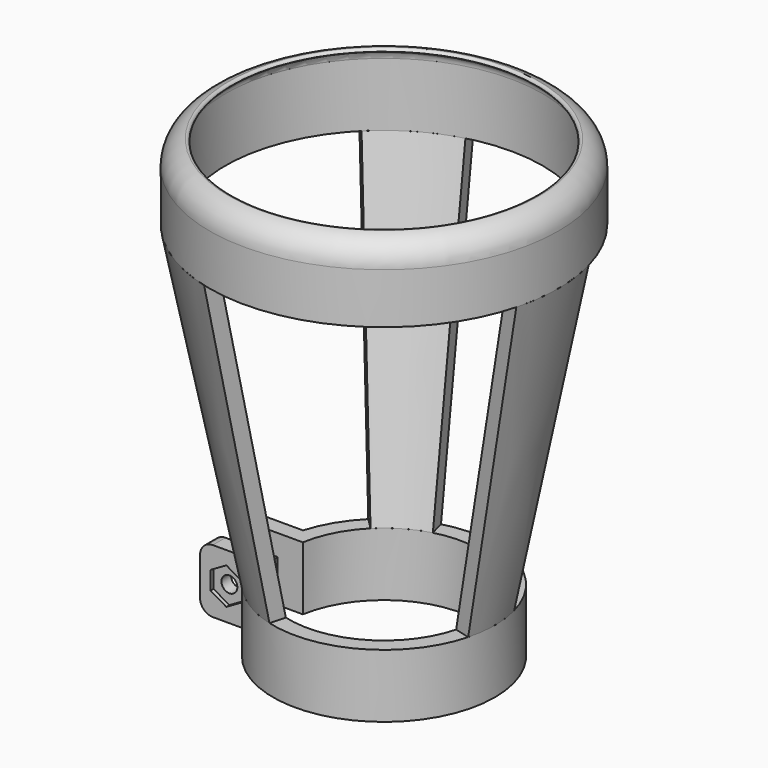
from build123d import *

# Parameters (mm, degrees)
F0_W           = 3.175
F0_H           = 12.7
F1_ANGLE_BACK  = 15
F1_ANGLE       = 30
F0_W_2         = 4.4764786097
F0_H_2         = 0.6337500702
F4_COUNT       = 3
F4_ANGLE       = 240
F0_W_3         = 7.0289915919
F5_DEPTH       = 6.35
F6_DEPTH       = 3.175
F8_D           = 3.175
F8_CBORE_D     = 6.35
F8_CBORE_DEPTH = 0.508
F9_R           = 1.5875
F10_DEPTH      = 0.762
F12_R          = 0.508


# Not quite as in the source:
# - a fillet or chamfer that OpenCascade refuses, or shapes differently, is made with other operations: its cross-section is extruded or revolved along the edge and cut away or added


with BuildPart() as f1:
    # F0 (on Front) → F1 (revolve)
    with BuildSketch(Plane.XZ, mode=Mode.PRIVATE) as f1_sk:
        with Locations((33.3375, 76.2)):
            Rectangle(F0_W, F0_H)
    revolve(f1_sk.sketch.rotate(Axis((0, 0, 38.1), (0, 0, -1)), -F1_ANGLE_BACK), axis=Axis((0, 0, 38.1), (0, 0, -1)), revolution_arc=F1_ANGLE)

    # F0 (on Front) → F3 (revolve)
    with BuildSketch(Plane.XZ):
        with Locations((33.3375, 76.2)):
            Rectangle(F0_W, F0_H)
        with BuildLine():
            ThreePointArc((30.4485213903, 84.3885183416), (31.3917014684, 83.6762766383), (31.75, 82.55))
            Line((31.75, 82.55), (34.925, 82.55))
            Line((34.925, 82.55), (34.925, 84.3885183416))
            Line((34.925, 84.3885183416), (30.4485213903, 84.3885183416))
        make_face()
        with Locations((32.6867606951, 84.7053933767)):
            Rectangle(F0_W_2, F0_H_2)
    revolve(axis=Axis((0, 0, 38.1), (0, 0, -1)))

    # F11: fillet of radius 5.08 on 1 edges, made by hand

    # F11_s1 → F11_t2 (revolve, cut)
    with BuildSketch(Plane.XZ):
        with BuildLine():
            ThreePointArc((30.4485213903, 85.0222684118), (33.6444926413, 83.3502269867), (34.925, 79.9782460158))
            Line((34.925, 79.9782460158), (34.925, 85.0222684118))
            Line((34.925, 85.0222684118), (30.4485213903, 85.0222684118))
        make_face()
    revolve(axis=Axis((0, 0, 85.0222684118), (0, 0, -1)), mode=Mode.SUBTRACT)

    # F12
    f12_edges = [f1.edges().sort_by_distance(p)[0] for p in [
        (-30.448521, 0, 85.022268),
    ]]
    fillet(f12_edges, radius=F12_R)


with BuildPart() as f1b:
    # F0 (on Front) → F1, piece 2 (revolve)
    with BuildSketch(Plane.XZ, mode=Mode.PRIVATE) as f1_sk:
        with Locations((20.6375, 0)):
            Rectangle(F0_W, F0_H)
    revolve(f1_sk.sketch.rotate(Axis((0, 0, 38.1), (0, 0, -1)), -F1_ANGLE_BACK), axis=Axis((0, 0, 38.1), (0, 0, -1)), revolution_arc=F1_ANGLE)

    # F0 (on Front) → F3, piece 2 (revolve)
    with BuildSketch(Plane.XZ):
        with Locations((20.6375, 0)):
            Rectangle(F0_W, F0_H)
    revolve(axis=Axis((0, 0, 38.1), (0, 0, -1)))

    # F0 (on Front) → F5 (join, symmetric)
    with BuildSketch(Plane.XZ):
        with BuildLine():
            Line((-29.21, -6.35), (-26.0789915919, -6.35))
            Line((-26.0789915919, -6.35), (-26.0789915919, 6.35))
            Line((-26.0789915919, 6.35), (-29.21, 6.35))
            ThreePointArc((-29.21, 6.35), (-31.0060512242, 5.6060512242), (-31.75, 3.81))
            Line((-31.75, 3.81), (-31.75, -3.81))
            ThreePointArc((-31.75, -3.81), (-31.0060512242, -5.6060512242), (-29.21, -6.35))
        make_face()
        with Locations((-22.564495796, 0)):
            Rectangle(F0_W_3, F0_H)
    extrude(amount=F5_DEPTH, both=True)

    # F0 (on Front) → F6 (cut, symmetric)
    with BuildSketch(Plane.XZ):
        Polygon((-19.05, 6.35), (-12.0210084081, 6.35), (-12.0210084081, 10.3498157114), (-26.0789915919, 10.3498157114), (-26.0789915919, 6.35), align=None)
        Polygon((-12.0210084081, -10.3498157114), (-12.0210084081, -6.35), (-19.05, -6.35), (-26.0789915919, -6.35), (-26.0789915919, -10.3498157114), align=None)
        with Locations((-15.535504204, 0)):
            Rectangle(F0_W_3, F0_H)
        with Locations((-22.564495796, 0)):
            Rectangle(F0_W_3, F0_H)
        with BuildLine():
            Line((-29.21, -6.35), (-26.0789915919, -6.35))
            Line((-26.0789915919, -6.35), (-26.0789915919, 6.35))
            Line((-26.0789915919, 6.35), (-29.21, 6.35))
            ThreePointArc((-29.21, 6.35), (-31.0060512242, 5.6060512242), (-31.75, 3.81))
            Line((-31.75, 3.81), (-31.75, -3.81))
            ThreePointArc((-31.75, -3.81), (-31.0060512242, -5.6060512242), (-29.21, -6.35))
        make_face()
    extrude(amount=F6_DEPTH, both=True, mode=Mode.SUBTRACT)

    # F8 (through all)
    with Locations(Plane(origin=(0, 6.35, 0), x_dir=(-1, 0, 0), z_dir=(0, 1, 0))):
        with Locations((26.4853648841, 0)):
            CounterBoreHole(F8_D / 2, F8_CBORE_D / 2, F8_CBORE_DEPTH)

    # F9 (on face) → F10 (cut)
    with BuildSketch(Plane.XZ.offset(6.35)):
        Polygon((-26.4853648841, -3.6661742094), (-23.3103648841, -1.8330871047), (-23.3103648841, 1.8330871047), (-26.4853648841, 3.6661742094), (-29.6603648841, 1.8330871047), (-29.6603648841, -1.8330871047), align=None)
        with Locations((-26.4853648841, 0)):
            Circle(F9_R, mode=Mode.SUBTRACT)
    extrude(amount=-F10_DEPTH, mode=Mode.SUBTRACT)


with BuildPart() as f2:
    # F1_face (on face) → F2 section 0
    with BuildSketch(Plane(origin=(32.9828951007, 0, 69.85), x_dir=(1, 0, 0), z_dir=(0, 0, -1))):
        with BuildLine():
            ThreePointArc((-2.3147501161, 8.217504682), (-1.2328951007, 0), (-2.3147501161, -8.217504682))
            Line((-2.3147501161, -8.217504682), (0.7520643824, -9.0392551502))
            ThreePointArc((0.7520643824, -9.0392551502), (1.9421048993, 0), (0.7520643824, 9.0392551502))
            Line((0.7520643824, 9.0392551502), (-2.3147501161, 8.217504682))
        make_face()
    # F1_face1 (on face) → F2 section 1
    with BuildSketch(Plane(origin=(20.4428029825, 0, 6.35), x_dir=(1, 0, 0), z_dir=(0, 0, 1))):
        with BuildLine():
            ThreePointArc((1.0248985068, -5.7522532774), (1.7821970175, 0), (1.0248985068, 5.7522532774))
            Line((1.0248985068, 5.7522532774), (-2.0419159917, 4.9305028092))
            ThreePointArc((-2.0419159917, 4.9305028092), (-1.3928029825, 0), (-2.0419159917, -4.9305028092))
            Line((-2.0419159917, -4.9305028092), (1.0248985068, -5.7522532774))
        make_face()
    loft()


with BuildPart() as f4_1:
    # F4: instance of F2
    add(f2.part.rotate(Axis((0, 0, 38.1), (0, 0, -1)), 1 * F4_ANGLE / (F4_COUNT - 1)))


with BuildPart() as f4_2:
    # F4: instance of F2
    add(f2.part.rotate(Axis((0, 0, 38.1), (0, 0, -1)), 2 * F4_ANGLE / (F4_COUNT - 1)))


solid = Compound([f1.part, f1b.part, f2.part, f4_1.part, f4_2.part])
